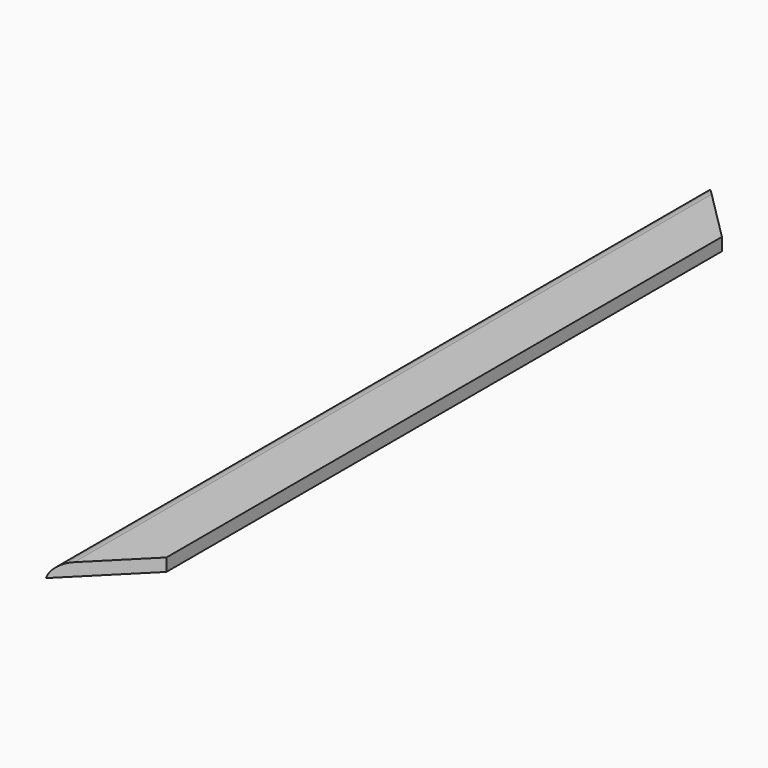
from build123d import *

# Parameters (mm, degrees)
F0_W        = 21
F0_H        = 260
F1_DEPTH    = 4
F3_DEPTH    = 4.001
F4_T1_DEPTH = 284.4948974279


# Not quite as in the source:
# - a fillet or chamfer that OpenCascade refuses, or shapes differently, is made with other operations: its cross-section is extruded or revolved along the edge and cut away or added


with BuildPart() as f1:
    # F0 (on Top) → F1 (new body)
    with BuildSketch(Plane.XY):
        Rectangle(F0_W, F0_H)
    extrude(amount=F1_DEPTH)

    # F2 (on face) → F3 (cut, through all)
    with BuildSketch(Plane.XY.offset(4)):
        Polygon((10.5, 130), (-10.5, 130), (10.5, 109), align=None)
        Polygon((10.5, -109), (-10.5, -130), (10.5, -130), align=None)
    extrude(amount=-F3_DEPTH, mode=Mode.SUBTRACT)

    # F4: fillet of radius 5 on 1 edges, made by hand

    # F4_s2 → F4_t1 (cut)
    with BuildSketch(Plane.XZ.offset(-142.2474487139)):
        with BuildLine():
            ThreePointArc((-5.6010205144, 4), (-8.7632981746, 2.8729833462), (-10.5, 0))
            Line((-10.5, 0), (-10.5, 4))
            Line((-10.5, 4), (-5.6010205144, 4))
        make_face()
    extrude(amount=F4_T1_DEPTH, mode=Mode.SUBTRACT)


solid = f1.part
